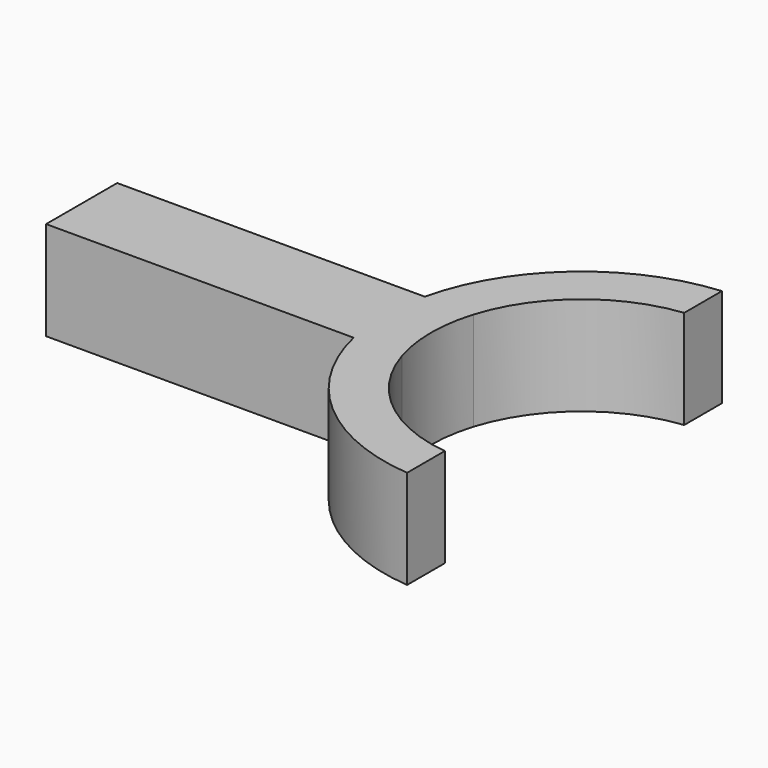
from build123d import *

# Parameters (mm, degrees)
F1_DEPTH = 20


# Not quite as in the source:
# - a feature names something its author has since deleted; it is built from what else it names


with BuildPart() as f1:
    # F0 (on Top) → F1 (new body)
    with BuildSketch(Plane.XY):
        with BuildLine():
            ThreePointArc((-29.1418942418, 9), (-19.4766119099, 23.471505885), (-3.470733695, 30.3018812554))
            Line((-3.470733695, 30.3018812554), (-3.470733695, 39.8491406133))
            ThreePointArc((-3.470733695, 39.8491406133), (-26.2357325621, 30.1941440834), (-38.9743505398, 9))
            Line((-38.9743505398, 9), (-29.1418942418, 9))
        make_face()
        with BuildLine():
            ThreePointArc((-29.1418942418, -9), (-30.5, 0), (-29.1418942418, 9))
            Line((-29.1418942418, 9), (-38.9743505398, 9))
            ThreePointArc((-38.9743505398, 9), (-40, 0), (-38.9743505398, -9))
            Line((-38.9743505398, -9), (-29.1418942418, -9))
        make_face()
        with BuildLine():
            ThreePointArc((-3.470733695, -30.3018812554), (-19.4766119099, -23.471505885), (-29.1418942418, -9))
            Line((-29.1418942418, -9), (-38.9743505398, -9))
            ThreePointArc((-38.9743505398, -9), (-26.2357325621, -30.1941440834), (-3.470733695, -39.8491406133))
            Line((-3.470733695, -39.8491406133), (-3.470733695, -30.3018812554))
        make_face()
        with BuildLine():
            ThreePointArc((-38.9743505398, -9), (-40, 0), (-38.9743505398, 9))
            Line((-38.9743505398, 9), (-101.2608483434, 9))
            Line((-101.2608483434, 9), (-101.2608483434, -9))
            Line((-101.2608483434, -9), (-38.9743505398, -9))
        make_face()
    extrude(amount=F1_DEPTH)


solid = f1.part
